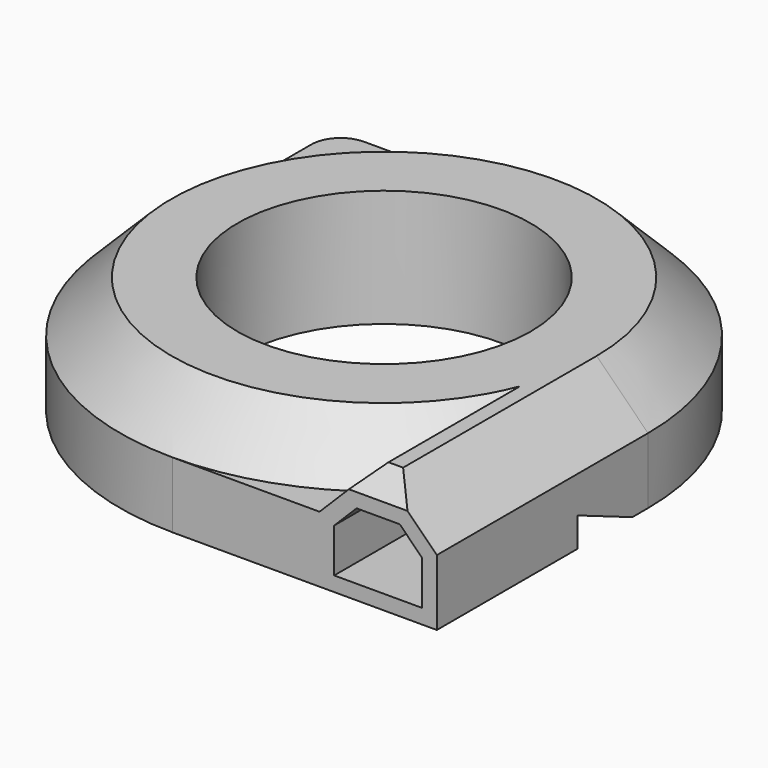
from build123d import *

# Parameters (mm, degrees)
F7_DEPTH       = 18
F8_ANGLE       = 270
F9_DEPTH       = 18
F15_DEPTH      = 6
F16_DEPTH      = 7
F16_DEPTH_BACK = 1
F17_T4_DEPTH   = 22.2867319519
F20_DEPTH      = 4.5
F19_R          = 1.5
F21_DEPTH      = 5
F23_W          = 11.0148127368
F23_H          = 3
F24_DEPTH      = 4.5
F25_SIZE       = 3.5
F26_SIZE       = 1.5


# Not quite as in the source:
# - a fillet or chamfer that OpenCascade refuses, or shapes differently, is made with other operations: its cross-section is extruded or revolved along the edge and cut away or added


with BuildPart() as f5:
    # F0 (on Front) → F5 (revolve)
    with BuildSketch(Plane.XZ):
        Polygon((10, 0), (18, 0), (18, 4.5), (14.5, 8), (10, 8), align=None)
    revolve(axis=Axis((0, 0, 0), (0, 0, 1)))

    # F1 (on Front) → F7 (join)
    with BuildSketch(Plane.XZ):
        Polygon((10, 0), (18, 0), (18, 4.5), (14.5, 8), (10, 8), align=None)
    extrude(amount=F7_DEPTH)


with BuildPart() as f8:
    # F2 (on Front) → F8 (revolve)
    with BuildSketch(Plane.XZ):
        Polygon((10.9985324027, 3.999999641), (11, 1), (17, 1), (17, 4), (14.0656156805, 7), align=None)
    revolve(axis=Axis((0, 0, 0), (0, 0, 1)), revolution_arc=F8_ANGLE)


with BuildPart() as f9:
    # F3 (on Front) → F9 (new body)
    with BuildSketch(Plane.XZ):
        Polygon((11, 4), (11, 1), (17, 1), (17, 4), (14, 7), align=None)
    extrude(amount=F9_DEPTH)


with BuildPart() as f5_1:
    add(f5.part)

    # F10: cut F8
    add(f8.part, mode=Mode.SUBTRACT)

    # F11: cut F9
    add(f9.part, mode=Mode.SUBTRACT)

    # F13 (on offset) → F15 (join)
    with BuildSketch(Plane.YZ.offset(11)):
        Polygon((-6, 7), (-18, 7), (-18, 5.5266313693), (-10, 3), (-6, 3), align=None)
    extrude(amount=F15_DEPTH)

    # F17: chamfer of 2 on 1 edges, made by hand


with BuildPart() as f16:
    # F14 (on offset) → F16 (new body, two sides)
    with BuildSketch(Plane.YZ.offset(11)) as f16_sk:
        Polygon((1, -1), (-6, 2), (-6, -1), align=None)
    extrude(amount=F16_DEPTH)
    extrude(f16_sk.sketch, amount=-F16_DEPTH_BACK)


with BuildPart() as f17_tool2:
    # F17_s3 → F17_t4 (new body)
    with BuildSketch(Plane.XZ.offset(0.8566340241)):
        Polygon((15, 7), (17, 5), (17, 7), align=None)
    extrude(amount=F17_T4_DEPTH)

    split(bisect_by=Plane(origin=(11.25, 0, 11.25), x_dir=(0, 1, 0), z_dir=(0.7071067812, 0, 0.7071067812)), keep=Keep.TOP)


with BuildPart() as f5_2:
    add(f5_1.part)

    # F17_t1: cut F17_tool2
    add(f17_tool2.part, mode=Mode.SUBTRACT)

    # F18: cut F16
    add(f16.part, mode=Mode.SUBTRACT)

    # F6 (on Top) → F20 (join)
    with BuildSketch(Plane.XY):
        with BuildLine():
            Line((-6, 16.8), (-14.8, 16.8))
            ThreePointArc((-14.8, 16.8), (-16.2142135624, 16.2142135624), (-16.8, 14.8))
            Line((-16.8, 14.8), (-16.8, 6))
            Line((-16.8, 6), (-6, 16.8))
        make_face()
    extrude(amount=F20_DEPTH)


with BuildPart() as f21:
    # F19 (on Top) → F21 (new body)
    with BuildSketch(Plane.XY):
        with Locations((-13.8, 13.8)):
            Circle(F19_R)
    extrude(amount=F21_DEPTH)


with BuildPart() as f5_3:
    add(f5_2.part)

    # F22: cut F21
    add(f21.part, mode=Mode.SUBTRACT)

    # F23 (on Top) → F24 (join)
    with BuildSketch(Plane.XY):
        with Locations((5.4925936316, -16.5)):
            Rectangle(F23_W, F23_H)
    extrude(amount=F24_DEPTH)

    # F25
    f25_edges = [f5_3.edges().sort_by_distance(p)[0] for p in [
        (10, -14.25, 8),
    ]]
    chamfer(f25_edges, length=F25_SIZE)

    # F26
    f26_edges = [f5_3.edges().sort_by_distance(p)[0] for p in [
        (14, -18, 8),
    ]]
    chamfer(f26_edges, length=F26_SIZE)


solid = f5_3.part
